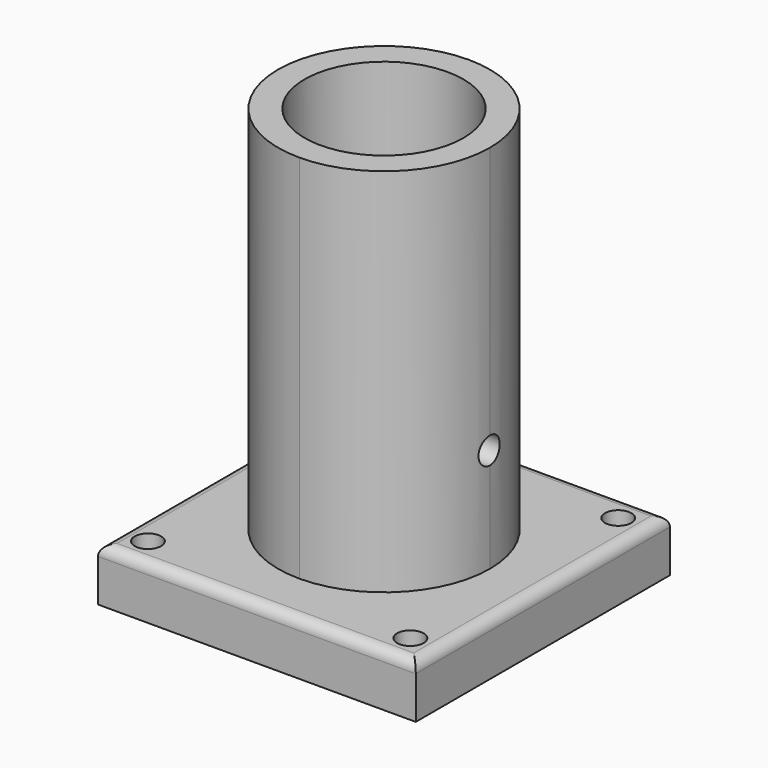
from build123d import *

# Parameters (mm, degrees)
F0_W        = 50.8
F0_H        = 50.8
F1_DEPTH    = 101.6
F0_W_2      = 76.2
F0_H_2      = 76.2
F0_R        = 3.175
F2_DEPTH    = 12.7
F3_R        = 19.05
F4_DEPTH    = 101.601
F5_R        = 3.175
F6_DEPTH    = 25.4
F7_T1_DEPTH = 88.9
F8_R        = 2.54


# Not quite as in the source:
# - a fillet or chamfer that OpenCascade refuses, or shapes differently, is made with other operations: its cross-section is extruded or revolved along the edge and cut away or added


with BuildPart() as f1:
    # F0 (on Top) → F1 (new body)
    with BuildSketch(Plane.XY):
        Rectangle(F0_W, F0_H)
    extrude(amount=F1_DEPTH)

    # F0 (on Top) → F2 (join)
    with BuildSketch(Plane.XY):
        Rectangle(F0_W_2, F0_H_2)
        with Locations((-31.6072627902, -31.269069761)):
            Circle(F0_R, mode=Mode.SUBTRACT)
        with Locations((31.3326152668, -31.2626581123)):
            Circle(F0_R, mode=Mode.SUBTRACT)
        Rectangle(F0_W, F0_H, mode=Mode.SUBTRACT)
        with Locations((-31.2740796408, 31.5370819021)):
            Circle(F0_R, mode=Mode.SUBTRACT)
        with Locations((31.2819033467, 31.1061042501)):
            Circle(F0_R, mode=Mode.SUBTRACT)
    extrude(amount=F2_DEPTH)

    # F3 (on face) → F4 (cut, through all)
    with BuildSketch(Plane.XY.offset(101.6)):
        Circle(F3_R)
    extrude(amount=-F4_DEPTH, mode=Mode.SUBTRACT)

    # F5 (on face) → F6 (cut)
    with BuildSketch(Plane.YZ.offset(25.4)):
        with Locations((0, 37.7008840442)):
            Circle(F5_R)
    extrude(amount=-F6_DEPTH, mode=Mode.SUBTRACT)

    # F7: fillet of radius 25.4 on 4 edges, made by hand

    # F7_s2 → F7_t1 (cut)
    with BuildSketch(Plane.XY.offset(12.7)):
        with BuildLine():
            ThreePointArc((0, -25.4), (17.9605122421, -17.9605122421), (25.4, 0))
            Line((25.4, 0), (25.908, 0))
            Line((25.908, 0), (25.908, -25.908))
            Line((25.908, -25.908), (0, -25.908))
            Line((0, -25.908), (0, -25.4))
        make_face()
        with BuildLine():
            ThreePointArc((25.4, 0), (17.9605122421, 17.9605122421), (0, 25.4))
            Line((0, 25.4), (0, 25.908))
            Line((0, 25.908), (25.908, 25.908))
            Line((25.908, 25.908), (25.908, 0))
            Line((25.908, 0), (25.4, 0))
        make_face()
        with BuildLine():
            ThreePointArc((0, -25.4), (-17.9605122421, -17.9605122421), (-25.4, 0))
            Line((-25.4, 0), (-25.908, 0))
            Line((-25.908, 0), (-25.908, -25.908))
            Line((-25.908, -25.908), (0, -25.908))
            Line((0, -25.908), (0, -25.4))
        make_face()
        with BuildLine():
            ThreePointArc((-25.4, 0), (-17.9605122421, 17.9605122421), (0, 25.4))
            Line((0, 25.4), (0, 25.908))
            Line((0, 25.908), (-25.908, 25.908))
            Line((-25.908, 25.908), (-25.908, 0))
            Line((-25.908, 0), (-25.4, 0))
        make_face()
    extrude(amount=F7_T1_DEPTH, mode=Mode.SUBTRACT)

    # F8
    f8_edges = [f1.edges().sort_by_distance(p)[0] for p in [
        (0, -38.1, 12.7),
        (38.1, 0, 12.7),
        (-38.1, 0, 12.7),
        (0, 38.1, 12.7),
    ]]
    fillet(f8_edges, radius=F8_R)


solid = f1.part
